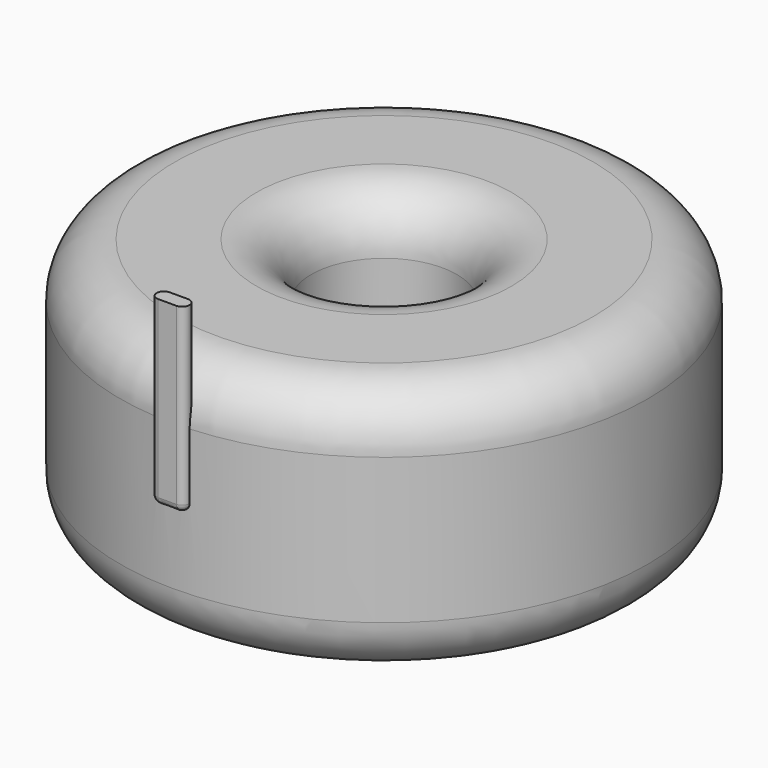
from build123d import *

# Parameters (mm, degrees)
F0_R     = 72.5
F0_R_2   = 20
F1_DEPTH = 35
F2_R     = 15
F4_DEPTH = 50
F5_R     = 1.9999


# Not quite as in the source:
# - a fillet or chamfer is up to 0.001 mm smaller than in the source, because OpenCascade refuses the exact size


with BuildPart() as f1:
    # F0 (on Top) → F1 (new body, symmetric)
    with BuildSketch(Plane.XY):
        Circle(F0_R)
        Circle(F0_R_2, mode=Mode.SUBTRACT)
    extrude(amount=F1_DEPTH, both=True)

    # F2
    f2_edges = [f1.edges().sort_by_distance(p)[0] for p in [
        (-20, 0, 35),
        (20, 0, 0),
        (-20, 0, -35),
        (-72.5, 0, -35),
        (72.5, 0, 0),
        (-72.5, 0, 35),
    ]]
    fillet(f2_edges, radius=F2_R)

    # F3 (on Top) → F4 (join)
    with BuildSketch(Plane.XY):
        with BuildLine():
            Line((2.5, -70.4568837309), (-2.5, -70.4568837309))
            ThreePointArc((-2.5, -70.4568837309), (-4.5, -72.4568837309), (-2.5, -74.4568837309))
            Line((-2.5, -74.4568837309), (2.5, -74.4568837309))
            ThreePointArc((2.5, -74.4568837309), (4.5, -72.4568837309), (2.5, -70.4568837309))
        make_face()
    extrude(amount=F4_DEPTH)

    # F5 (radius 2 in the source; OpenCascade refuses exactly that, so slightly less here)
    f5_edges = [f1.edges().sort_by_distance(p)[0] for p in [
        (0, -74.456884, 0),
    ]]
    fillet(f5_edges, radius=F5_R)


solid = f1.part
